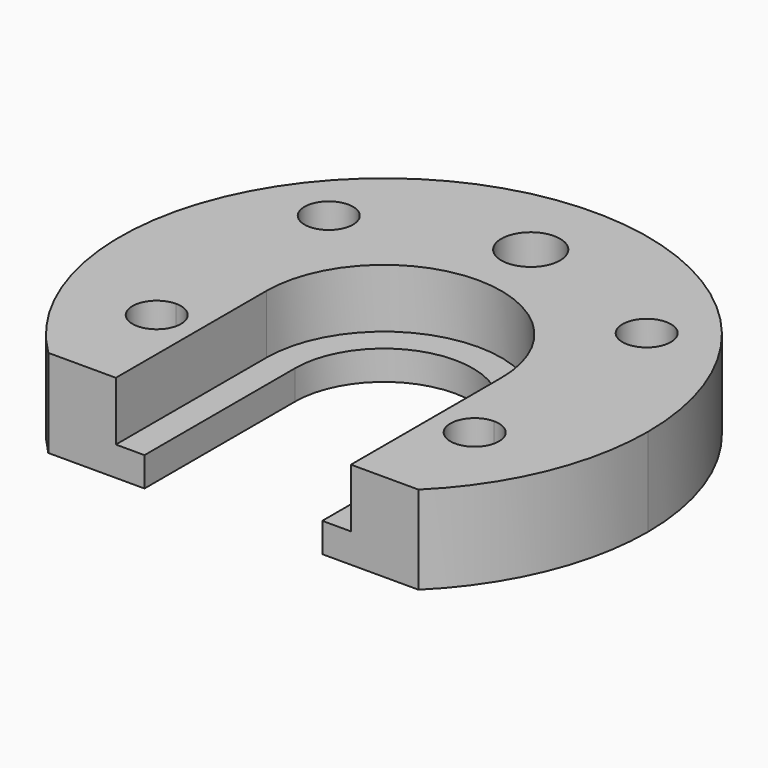
from build123d import *

# Parameters (mm, degrees)
F1_DEPTH = 6
F2_R     = 2
F3_DEPTH = 25.4
F5_DEPTH = 4


with BuildPart() as f1:
    # F0 (on Top) → F1 (new body)
    with BuildSketch(Plane.XY):
        with BuildLine():
            ThreePointArc((12.5979084153, -12.807573094), (16.5689868381, -6.9433349451), (17.965, 0))
            ThreePointArc((17.965, 0), (-6.9433349451, 16.5689868381), (-12.5979084153, -12.807573094))
            Line((-12.5979084153, -12.807573094), (-6.05, -12.807573094))
            Line((-6.05, -12.807573094), (-6.05, 0))
            ThreePointArc((-6.05, 0), (0, 6.05), (6.05, 0))
            Line((6.05, 0), (6.05, -12.807573094))
            Line((6.05, -12.807573094), (12.5979084153, -12.807573094))
        make_face()
    extrude(amount=F1_DEPTH)

    # F2 (on face) → F3 (cut)
    with BuildSketch(Plane.XY.offset(6)):
        with Locations((0, 12.49)):
            Circle(F2_R)
        with BuildLine():
            ThreePointArc((-10.82, 7.1820178571), (-9.653273811, 7.6652916681), (-9.17, 8.8320178571))
            ThreePointArc((-9.17, 8.8320178571), (-11.986726189, 9.998744046), (-10.82, 7.1820178571))
        make_face()
        with BuildLine():
            ThreePointArc((-9.17, -5.8029047803), (-9.653273811, -4.6361785914), (-10.82, -4.1529047803))
            ThreePointArc((-10.82, -4.1529047803), (-11.986726189, -6.9696309693), (-9.17, -5.8029047803))
        make_face()
        with BuildLine():
            ThreePointArc((10.82, 7.1820178571), (11.986726189, 7.6652916681), (12.47, 8.8320178571))
            ThreePointArc((12.47, 8.8320178571), (9.653273811, 9.998744046), (10.82, 7.1820178571))
        make_face()
        with BuildLine():
            ThreePointArc((12.47, -5.8029047803), (11.986726189, -4.6361785914), (10.82, -4.1529047803))
            ThreePointArc((10.82, -4.1529047803), (9.653273811, -6.9696309693), (12.47, -5.8029047803))
        make_face()
    extrude(amount=-F3_DEPTH, mode=Mode.SUBTRACT)

    # F4 (on face) → F5 (cut)
    with BuildSketch(Plane.XY.offset(6)):
        with BuildLine():
            ThreePointArc((6.05, -5.2342621256), (7.4966659256, -2.7928480088), (8, 0))
            ThreePointArc((8, 0), (0, 8), (-8, 0))
            ThreePointArc((-8, 0), (-7.4966659256, -2.7928480088), (-6.05, -5.2342621256))
            Line((-6.05, -5.2342621256), (-6.05, 0))
            ThreePointArc((-6.05, 0), (0, 6.05), (6.05, 0))
            Line((6.05, 0), (6.05, -5.2342621256))
        make_face()
        with BuildLine():
            Line((8, -12.807573094), (8, 0))
            ThreePointArc((8, 0), (7.4966659256, -2.7928480088), (6.05, -5.2342621256))
            Line((6.05, -5.2342621256), (6.05, -12.807573094))
            Line((6.05, -12.807573094), (8, -12.807573094))
        make_face()
        with BuildLine():
            ThreePointArc((-6.05, -5.2342621256), (-7.4966659256, -2.7928480088), (-8, 0))
            Line((-8, 0), (-8, -12.807573094))
            Line((-8, -12.807573094), (-6.05, -12.807573094))
            Line((-6.05, -12.807573094), (-6.05, -5.2342621256))
        make_face()
        with BuildLine():
            ThreePointArc((-6.05, -5.2342621256), (0, -8), (6.05, -5.2342621256))
            Line((6.05, -5.2342621256), (6.05, 0))
            ThreePointArc((6.05, 0), (0, 6.05), (-6.05, 0))
            Line((-6.05, 0), (-6.05, -5.2342621256))
        make_face()
    extrude(amount=-F5_DEPTH, mode=Mode.SUBTRACT)


solid = f1.part
